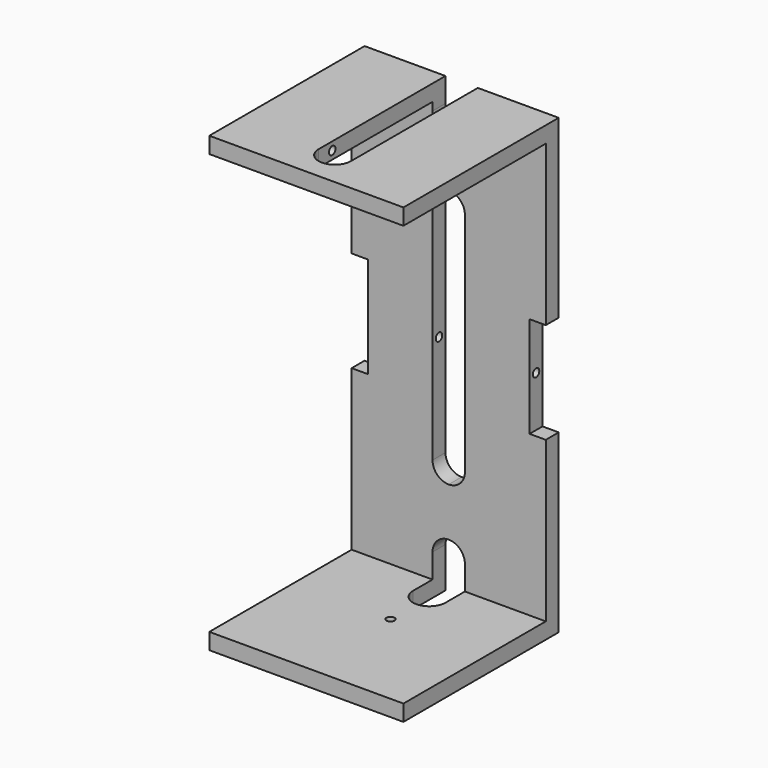
from build123d import *

# Parameters (mm, degrees)
F0_W            = 31.75
F0_H            = 6.35
F0_W_2          = 12.7
F0_H_2          = 101.6
F1_DEPTH        = 6.35
F2_DEPTH        = 76.2
F3_W            = 12.7
F3_H            = 68.58
F4_DEPTH        = 6.35
F5_W            = 12.7
F5_H            = 22.225
F6_DEPTH        = 6.35
F7_D            = 1.5875
F7_CSINK_D      = 3.175
F7_CSINK_ANGLE  = 90
F8_R            = 6.34999
F10_D           = 3.175
F12_D           = 3.175
F12_CSINK_D     = 6.35
F12_CSINK_ANGLE = 90
F13_R           = 1.5875
F14_DEPTH       = 12.7


# Not quite as in the source:
# - a fillet or chamfer is up to 0.001 mm smaller than in the source, because OpenCascade refuses the exact size


with BuildPart() as f1:
    # F0 (on Front) → F1 (new body)
    with BuildSketch(Plane.XZ):
        with Locations((-22.225, 174.625)):
            Rectangle(F0_W, F0_H)
        with Locations((22.225, 174.625)):
            Rectangle(F0_W, F0_H)
        with Locations((-22.225, 3.175)):
            Rectangle(F0_W, F0_H)
        with Locations((22.225, 3.175)):
            Rectangle(F0_W, F0_H)
        Polygon((-6.35, 171.45), (-38.1, 171.45), (-38.1, 108.712), (-31.75, 108.712), (-31.75, 69.088), (-38.1, 69.088), (-38.1, 6.35), (-6.35, 6.35), (-6.35, 22.225), (6.35, 22.225), (6.35, 6.35), (38.1, 6.35), (38.1, 69.088), (31.75, 69.088), (31.75, 108.712), (38.1, 108.712), (38.1, 171.45), (6.35, 171.45), (6.35, 161.925), (-6.35, 161.925), align=None)
        with Locations((0, 92.075)):
            Rectangle(F0_W_2, F0_H_2, mode=Mode.SUBTRACT)
    extrude(amount=F1_DEPTH)

    # F0 (on Front) → F2 (join)
    with BuildSketch(Plane.XZ):
        with Locations((-22.225, 174.625)):
            Rectangle(F0_W, F0_H)
        with Locations((22.225, 174.625)):
            Rectangle(F0_W, F0_H)
        with Locations((-22.225, 3.175)):
            Rectangle(F0_W, F0_H)
        with Locations((22.225, 3.175)):
            Rectangle(F0_W, F0_H)
        with Locations((0, 3.175)):
            Rectangle(F0_W_2, F0_H)
        with Locations((0, 174.625)):
            Rectangle(F0_W_2, F0_H)
    extrude(amount=F2_DEPTH)

    # F3 (on face) → F4 (cut, through all)
    with BuildSketch(Plane.XY.offset(177.8)):
        with Locations((0, -34.29)):
            Rectangle(F3_W, F3_H)
    extrude(amount=-F4_DEPTH, mode=Mode.SUBTRACT)

    # F5 (on face) → F6 (cut, through all)
    with BuildSketch(Plane(origin=(0, 0, 0), x_dir=(1, 0, 0), z_dir=(0, 0, -1))):
        with Locations((0, 11.1125)):
            Rectangle(F5_W, F5_H)
    extrude(amount=-F6_DEPTH, mode=Mode.SUBTRACT)

    # F7 (through all)
    with Locations(Plane(origin=(0, 0, 0), x_dir=(1, 0, 0), z_dir=(0, 1, 0))):
        with Locations((-3.175, -158.75), (3.175, -158.75)):
            CounterSinkHole(F7_D / 2, F7_CSINK_D / 2, counter_sink_angle=F7_CSINK_ANGLE)

    # F8 (radius 6.35 in the source; OpenCascade refuses exactly that, so slightly less here)
    f8_edges = [f1.edges().sort_by_distance(p)[0] for p in [
        (-6.35, -3.175, 22.225),
        (6.35, -3.175, 22.225),
        (-6.35, -3.175, 161.925),
        (6.35, -3.175, 161.925),
        (-6.35, -68.58, 174.625),
        (6.35, -68.58, 174.625),
        (6.35, -22.225, 3.175),
        (-6.35, -22.225, 3.175),
        (-6.35, -3.175, 41.275),
        (6.35, -3.175, 41.275),
        (-6.35, -3.175, 142.875),
        (6.35, -3.175, 142.875),
    ]]
    fillet(f8_edges, radius=F8_R)

    # F10 (through all)
    with Locations(Plane.YZ.offset(38.1)):
        with Locations((-3.175, 88.9)):
            Hole(F10_D / 2)

    # F12 (through all)
    with Locations(Plane(origin=(0, 0, 0), x_dir=(1, 0, 0), z_dir=(0, 0, -1))):
        with Locations((0, 34.925)):
            CounterSinkHole(F12_D / 2, F12_CSINK_D / 2, counter_sink_angle=F12_CSINK_ANGLE)

    # F13 (on Right) → F14 (cut, symmetric)
    with BuildSketch(Plane.YZ):
        with Locations((-55.5625, 174.625)):
            Circle(F13_R)
    extrude(amount=F14_DEPTH, both=True, mode=Mode.SUBTRACT)


solid = f1.part
